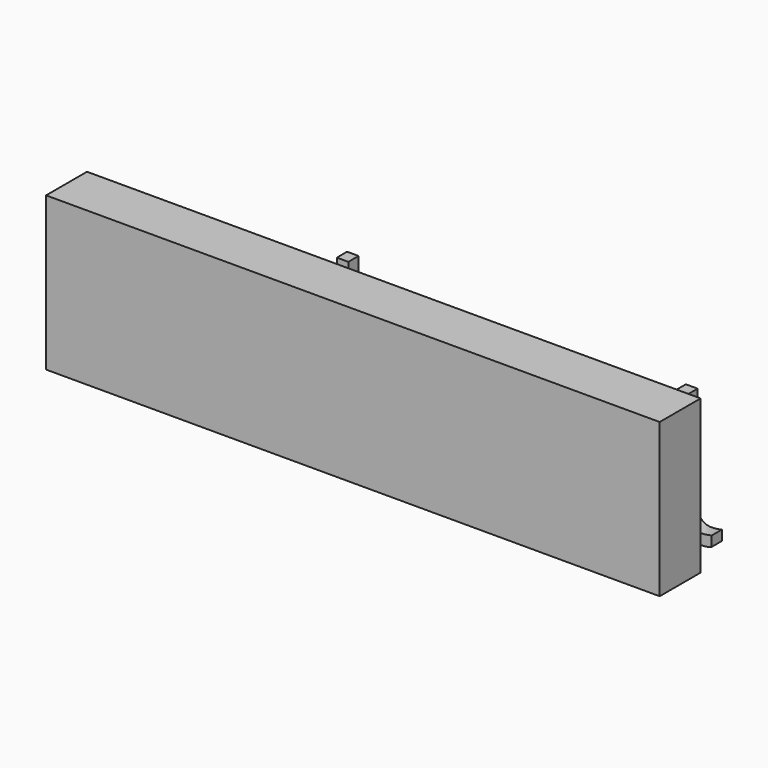
from build123d import *

# Parameters (mm, degrees)
F0_W         = 152.4
F0_H         = 50.8
F1_DEPTH     = 25.4
F3_W         = 25.4
F3_H         = 50.8
F4_DEPTH     = 152.4
F5_DEPTH     = 25.4
F2_TEXT_SIZE = 70.5555555556
F6_DEPTH     = 6.35


# Not quite as in the source:
# - Text() gives the source's letters only with a copy of the font that has no kerning and outlines rounded to 1/6400 em; it was checked with that copy


with BuildPart() as f1:
    # F0 (on Front) → F1 (new body)
    with BuildSketch(Plane.XZ):
        with Locations((-0.2342909575, 7.9074850983)):
            Rectangle(F0_W, F0_H)
    extrude(amount=F1_DEPTH)

    # F3 (on face) → F4 (join)
    with BuildSketch(Plane(origin=(-76.4342909575, 0, 0), x_dir=(0, -1, 0), z_dir=(-1, 0, 0))):
        with Locations((12.7, 7.9074850983)):
            Rectangle(F3_W, F3_H)
    extrude(amount=F4_DEPTH)

    # F5 (add): a face of the model
    f5_faces = [f1.faces().sort_by_distance(p)[0] for p in [
        (-76.4342909575, -12.7, -17.4925149017),
    ]]
    extrude(f5_faces, amount=F5_DEPTH)

    # F2 (on face) → F6 (join)
    with BuildSketch(Plane(origin=(0, 0, 0), x_dir=(-1, 0, 0), z_dir=(0, 1, 0))):
        with Locations((-75.9657090425, -17.4925149017)):
            Text('Jonathan', F2_TEXT_SIZE, font='Open Sans', text_align=(TextAlign.LEFT, TextAlign.BOTTOM))
    extrude(amount=F6_DEPTH)


solid = f1.part
